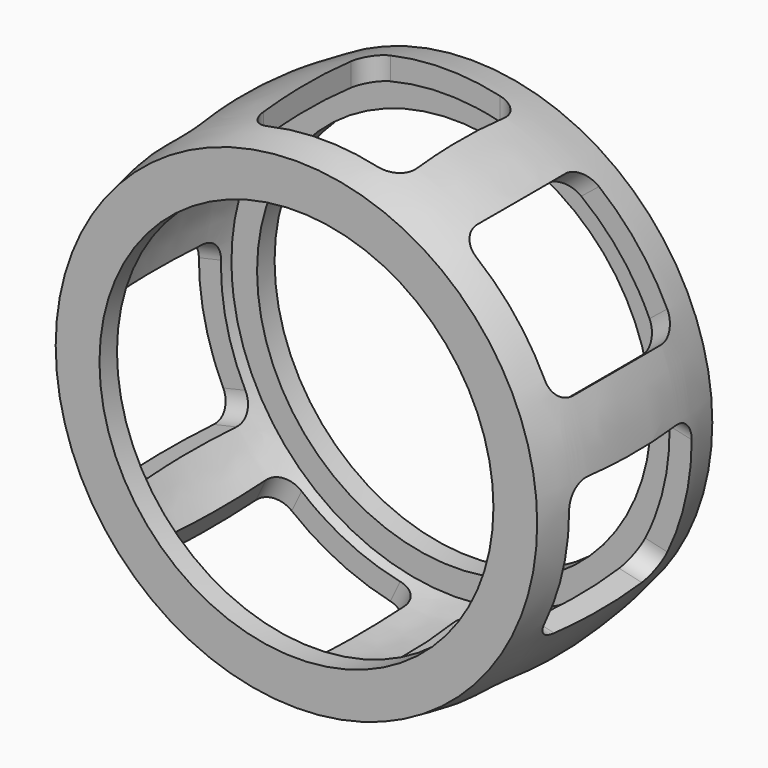
from build123d import *

# Parameters (mm, degrees)
F2_T            = -1
F4_DEPTH        = 11.5061026722
F4_COPIES_COUNT = 7


# Not quite as in the source:
# - a pattern or mirror of a feature is missing from the dataset's text; its kind, count and spacing are read off the source's solid


with BuildPart() as f1:
    # F0 (on Top) → F1 (revolve)
    with BuildSketch(Plane.XY):
        with BuildLine():
            Line((-9, -5), (-9, 5))
            Line((-9, 5), (-11, 5))
            ThreePointArc((-11, 5), (-11.5051025722, 0), (-11, -5))
            Line((-11, -5), (-9, -5))
        make_face()
    revolve(axis=Axis((0, -9.48, 0), (0, -1, 0)))

    # F2
    f2_openings = [f1.faces().sort_by_distance(p)[0] for p in [
        (9, 0, 0),
    ]]
    offset(amount=F2_T, openings=f2_openings, kind=Kind.INTERSECTION)

    # F3 (on Top) → F4 (cut, through all)
    with BuildSketch(Plane.XY):
        with BuildLine():
            Line((2.5, 3.5), (-2.5, 3.5))
            ThreePointArc((-2.5, 3.5), (-3.2071067812, 3.2071067812), (-3.5, 2.5))
            Line((-3.5, 2.5), (-3.5, -2.5))
            ThreePointArc((-3.5, -2.5), (-3.2071067812, -3.2071067812), (-2.5, -3.5))
            Line((-2.5, -3.5), (0, -3.5))
            Line((0, -3.5), (2.5, -3.5))
            ThreePointArc((2.5, -3.5), (3.2071067812, -3.2071067812), (3.5, -2.5))
            Line((3.5, -2.5), (3.5, 2.5))
            ThreePointArc((3.5, 2.5), (3.2071067812, 3.2071067812), (2.5, 3.5))
        make_face()
    f4 = extrude(amount=F4_DEPTH, mode=Mode.SUBTRACT)

    # F4_copies: F4 ×7 about axis
    f4_copies_axis = Axis((0, 0, 0), (0, 1, 0))
    for i in range(1, F4_COPIES_COUNT):
        add(f4.rotate(f4_copies_axis, i * 360 / F4_COPIES_COUNT), mode=Mode.SUBTRACT)


solid = f1.part
